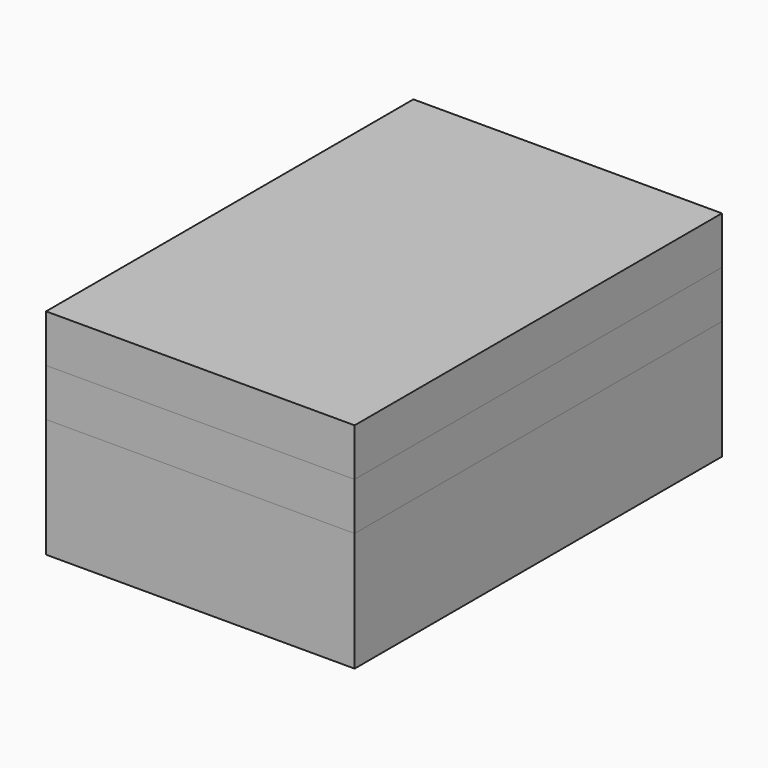
from build123d import *

# Parameters (mm, degrees)
F0_W     = 16.462284606
F0_H     = 24.4974466041
F1_DEPTH = 6.35
F2_W     = 16.462284606
F2_H     = 24.4974466041
F3_DEPTH = 2.54
F4_W     = 6.493705092
F4_H     = 3.0464301817
F5_DEPTH = 2.54
F6_W     = 16.462284606
F6_H     = 24.4974466041
F7_DEPTH = 2.54


# Not quite as in the source:
# - a feature names something its author has since deleted; it is built from what else it names


with BuildPart() as f1:
    # F0 (on Top) → F1 (new body)
    with BuildSketch(Plane.XY):
        with Locations((0.2442786936, 0.227171462)):
            Rectangle(F0_W, F0_H)
    extrude(amount=F1_DEPTH)


with BuildPart() as f3:
    # F2 (on face) → F3 (new body)
    with BuildSketch(Plane.XY.offset(6.35)):
        with Locations((0.2442786936, 0.227171462)):
            Rectangle(F2_W, F2_H)
    extrude(amount=F3_DEPTH)

    # F4 (on face) → F5 (cut)
    with BuildSketch(Plane.XY.offset(8.89)):
        with Locations((0.4903447116, 6.1370439362)):
            Rectangle(F4_W, F4_H)
    extrude(amount=-F5_DEPTH, mode=Mode.SUBTRACT)


with BuildPart() as f7:
    # F6 (on face) → F7 (new body)
    with BuildSketch(Plane.XY.offset(8.89)):
        with Locations((0.2442786936, 0.227171462)):
            Rectangle(F6_W, F6_H)
    extrude(amount=F7_DEPTH)


solid = Compound([f1.part, f3.part, f7.part])
